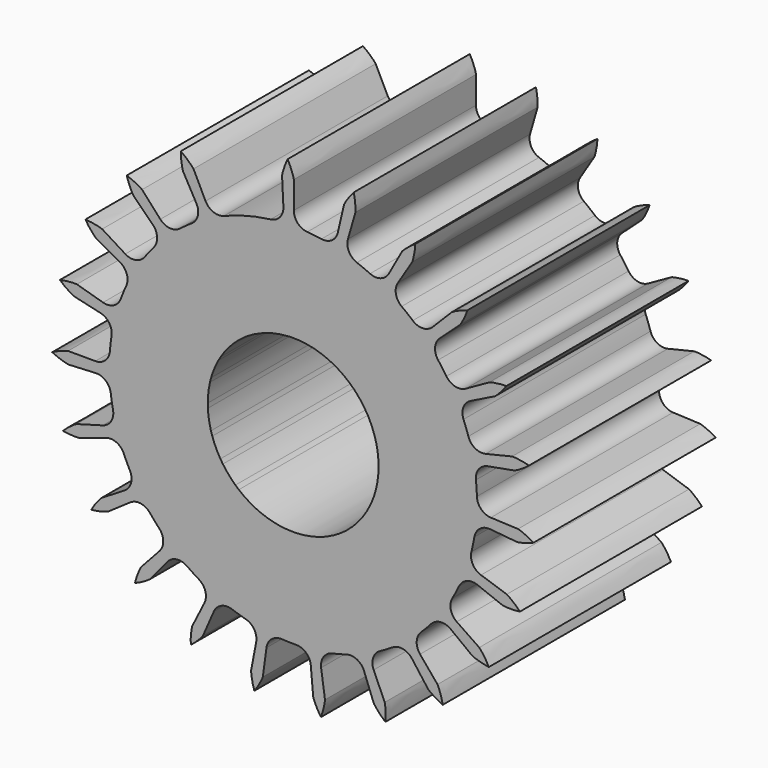
from build123d import *

# Parameters (mm, degrees)
F3_DEPTH        = 3.175
F3_COPIES_COUNT = 22
F3_COPIES_ANGLE = 333.5304
F4_R            = 0.2032


# Not quite as in the source:
# - a feature of the source that left no trace in its solid (it failed there, or was rolled back) is left out
# - a pattern or mirror of a feature is missing from the dataset's text; its kind, count and spacing are read off the source's solid


with BuildPart() as f3:
    # F2 (on Front) → F3 (new body)
    with BuildSketch(Plane.XZ):
        with BuildLine():
            add(Edge.make_bspline(
                [(-0.077612078, 3.3592404383), (-0.0703844716, 3.3458627043), (-0.050261849, 3.3073539493), (-0.0262314445, 3.2548922221), (0.0023217415, 3.1704242627), (-0.0031871923, 3.1867211618), (0.01005916, 3.1380066115)],
                knots=[0.569715009, 0.569715009, 0.569715009, 0.569715009, 0.6395714738, 0.772859937, 0.8935199848, 1, 1, 1, 1], degree=3))
            add(Edge.make_bspline(
                [(-0.077612078, 3.3592404383), (-0.0842141422, 3.3455431828), (-0.102536826, 3.3061461854), (-0.1241187255, 3.252630629), (-0.1487404219, 3.166934114), (-0.1439900135, 3.1834680456), (-0.1549724252, 3.1341937126)],
                knots=[0.569715009, 0.569715009, 0.569715009, 0.569715009, 0.6395714738, 0.772859937, 0.8935199848, 1, 1, 1, 1], degree=3))
            Line((-0.1549724252, 3.1341937126), (-0.126562572, 2.5596270889))
            ThreePointArc((-0.126562572, 2.5596270889), (-0.0591942181, 2.5620704446), (0.0082150948, 2.5627409996))
            Line((0.0082150948, 2.5627409996), (0.01005916, 3.1380066115))
        make_face()
        with BuildLine():
            Line((0.003816635, 1.1906188827), (0.0082150948, 2.5627409996))
            ThreePointArc((0.0082150948, 2.5627409996), (-0.0591942181, 2.5620704446), (-0.126562572, 2.5596270889))
            Line((-0.126562572, 2.5596270889), (-0.0587994605, 1.189172197))
            ThreePointArc((-0.0587994605, 1.189172197), (-0.0275009272, 1.1903073509), (0.003816635, 1.1906188827))
        make_face()
        with BuildLine():
            ThreePointArc((2.5627541667, 0), (1.8150430005, 1.8092340438), (0.0082150948, 2.5627409996))
            Line((0.0082150948, 2.5627409996), (0.003816635, 1.1906188827))
            ThreePointArc((0.003816635, 1.1906188827), (0.8432473159, 0.840548544), (1.190625, 0))
            ThreePointArc((1.190625, 0), (-0.8208470573, -0.8624372436), (-0.0587994605, 1.189172197))
            Line((-0.0587994605, 1.189172197), (-0.126562572, 2.5596270889))
            ThreePointArc((-0.126562572, 2.5596270889), (-1.7668276882, -1.8563482536), (2.5627541667, 0))
        make_face()
    extrude(amount=F3_DEPTH)

    # F3_copies: F3 ×22 about axis
    f3_copies_axis = Axis((0, 0, 0), (0, 1, 0))


with BuildPart() as f3_1:
    add(f3.part)
    for i in range(1, F3_COPIES_COUNT):
        add(f3.part.rotate(f3_copies_axis, i * F3_COPIES_ANGLE / (F3_COPIES_COUNT - 1)))

    # F4
    f4_edges = [f3_1.edges().sort_by_distance(p)[0] for p in [
        (-0.126563, -1.5875, 2.559627),
        (-1.134918, -1.5875, 2.297753),
        (-1.25418, -1.5875, 2.234892),
        (-1.720405, -1.5875, 1.899451),
        (-1.817911, -1.5875, 1.806352),
        (-2.17454, -1.5875, 1.356128),
        (-2.242846, -1.5875, 1.239899),
        (-2.462651, -1.5875, 0.709265),
        (-2.496542, -1.5875, 0.578781),
        (-2.562741, -1.5875, 0.008251),
        (-2.559629, -1.5875, -0.126527),
        (-2.467167, -1.5875, -0.693393),
        (-2.42729, -1.5875, -0.822174),
        (-2.183228, -1.5875, -1.342098),
        (-2.10963, -1.5875, -1.45505),
        (-1.7326, -1.5875, -1.888334),
        (-1.630901, -1.5875, -1.976833),
        (-1.14969, -1.5875, -2.290398),
        (-1.027655, -1.5875, -2.347687),
        (-0.479002, -1.5875, -2.517591),
        (-0.345948, -1.5875, -2.539297),
        (0.228257, -1.5875, -2.552569),
        (0.362172, -1.5875, -2.537034),
        (0.918089, -1.5875, -2.39266),
        (1.042641, -1.5875, -2.34107),
        (1.537826, -1.5875, -2.050074),
        (1.643505, -1.5875, -1.966368),
        (2.040151, -1.5875, -1.550966),
        (2.118888, -1.5875, -1.441535),
        (2.386712, -1.5875, -0.933443),
        (2.432496, -1.5875, -0.806642),
        (2.55105, -1.5875, -0.244653),
        (2.560385, -1.5875, -0.110163),
        (2.520617, -1.5875, 0.462817),
        (2.492791, -1.5875, 0.594728),
        (2.297737, -1.5875, 1.134951),
        (2.234875, -1.5875, 1.254211),
        (1.899427, -1.5875, 1.720432),
        (1.806327, -1.5875, 1.817936),
        (1.356097, -1.5875, 2.174559),
        (1.239868, -1.5875, 2.242863),
        (0.709231, -1.5875, 2.462661),
        (0.578746, -1.5875, 2.49655),
        (0.008215, -1.5875, 2.562741),
    ]]
    fillet(f4_edges, radius=F4_R)


solid = f3_1.part
